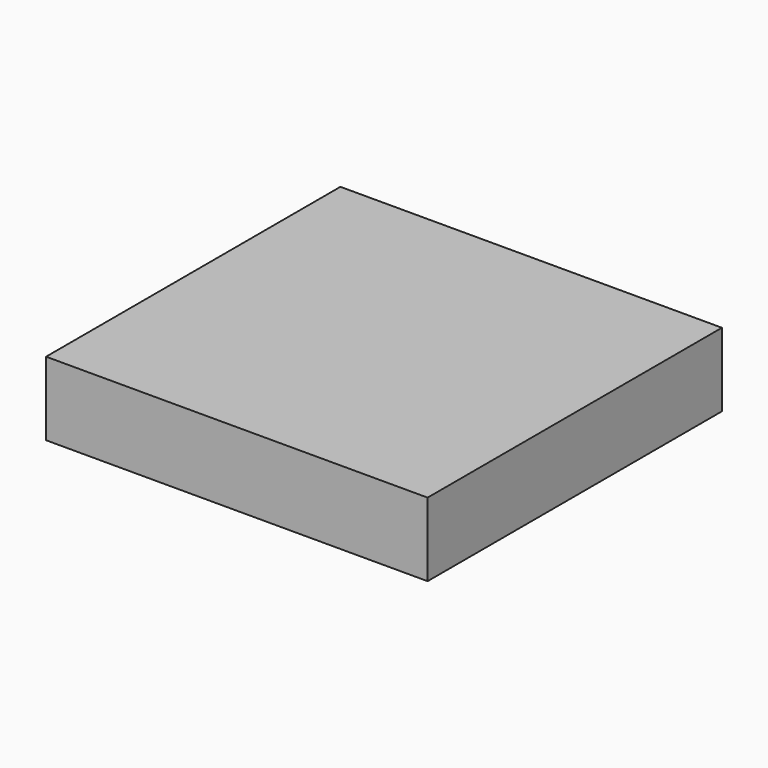
from build123d import *

# Parameters (mm, degrees)
F2_W     = 105.3663045168
F2_H     = 20.3218907118
F3_DEPTH = 101.6


# Not quite as in the source:
# - the program builds the solid bodies; features that only make, move or delete a surface that nothing else refers to are left out


with BuildPart() as f3:
    # F2 (on Front) → F3 (new body)
    with BuildSketch(Plane.XZ):
        with Locations((5.2134469151, -44.9923500419)):
            Rectangle(F2_W, F2_H)
    extrude(amount=F3_DEPTH)


solid = f3.part
